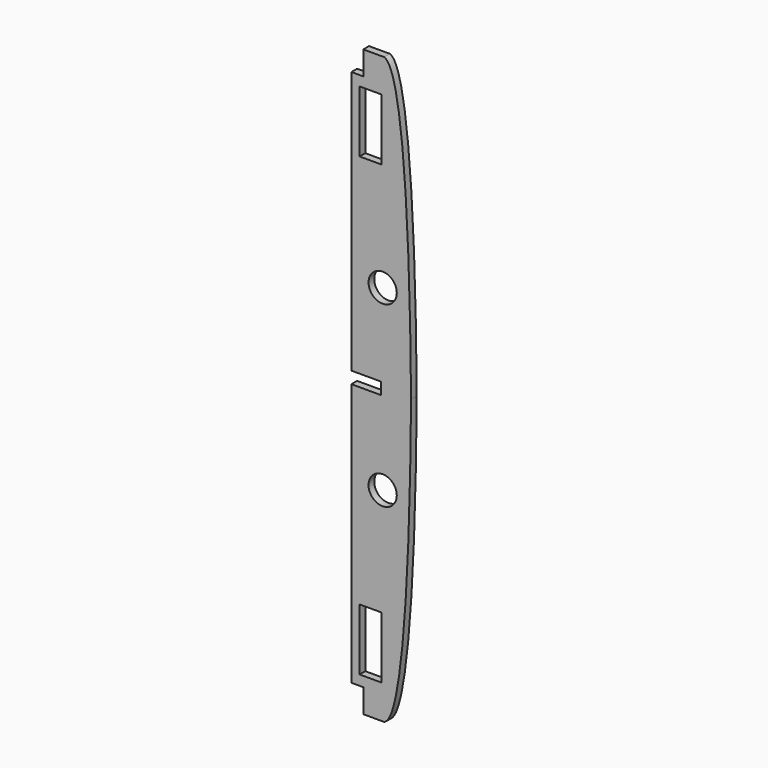
from build123d import *

# Parameters (mm, degrees)
F0_W     = 18.5761749744
F0_H     = 51.8475696445
F0_R     = 11.8720680475
F1_DEPTH = 6


# Not quite as in the source:
# - ends of sketch curves that miss each other by under 0.0002 mm in the source are joined
# - a feature names something its author has since deleted; it is built from what else it names


with BuildPart() as f1:
    # F0 (on Front) → F1 (new body)
    with BuildSketch(Plane.XZ):
        with BuildLine():
            add(Edge.make_bspline(
                [(192.7526748574, -288.1484243559), (215.2837565712, -280.7484243098), (215.2837563696, -43.999011342), (215.2526721504, -42.1484243381)],
                knots=[0, 0, 0, 0, 247.0268201774, 247.0268201774, 247.0268201774, 247.0268201774], degree=3))
            Line((215.2526721504, -42.1484243381), (190.2526734349, -42.1484243613))
            Line((190.2526734349, -42.1484243613), (190.2526734349, -47.1484243613))
            Line((190.2526734349, -47.1484243613), (165.2526734349, -47.1484243613))
            Line((165.2526734349, -47.1484243613), (165.2526734349, -268.1484243613))
            Line((165.2526734349, -268.1484243613), (175.2526734349, -268.1484243613))
            Line((175.2526734349, -268.1484243613), (175.2526734349, -288.1484243613))
            Line((175.2526734349, -288.1484243613), (192.7526748574, -288.1484243559))
        make_face()
        with Locations((181.4437263322, -233.8176692815)):
            Rectangle(F0_W, F0_H, mode=Mode.SUBTRACT)
        with Locations((191.5265821529, -117.0901346)):
            Circle(F0_R, mode=Mode.SUBTRACT)
        with BuildLine():
            add(Edge.make_bspline(
                [(192.7526744386, 203.8515756413), (215.2837561649, 196.4515756336), (215.2837563665, -40.2978373342), (215.2526721504, -42.1484243381)],
                knots=[0, 0, 0, 0, 247.0268201774, 247.0268201774, 247.0268201774, 247.0268201774], degree=3))
            Line((192.7526744386, 203.8515756413), (175.2526734349, 203.8515756387))
            Line((175.2526734349, 203.8515756387), (175.2526734349, 183.8515756387))
            Line((175.2526734349, 183.8515756387), (165.2526734349, 183.8515756387))
            Line((165.2526734349, 183.8515756387), (165.2526734349, -37.1484243613))
            Line((165.2526734349, -37.1484243613), (190.2526734349, -37.1484243613))
            Line((190.2526734349, -37.1484243613), (190.2526734349, -42.1484243613))
            Line((190.2526734349, -42.1484243613), (215.2526721504, -42.1484243381))
        make_face()
        with Locations((181.4437263322, 149.5208205589)):
            Rectangle(F0_W, F0_H, mode=Mode.SUBTRACT)
        with Locations((191.5265821529, 32.7932858774)):
            Circle(F0_R, mode=Mode.SUBTRACT)
    extrude(amount=F1_DEPTH)


solid = f1.part
